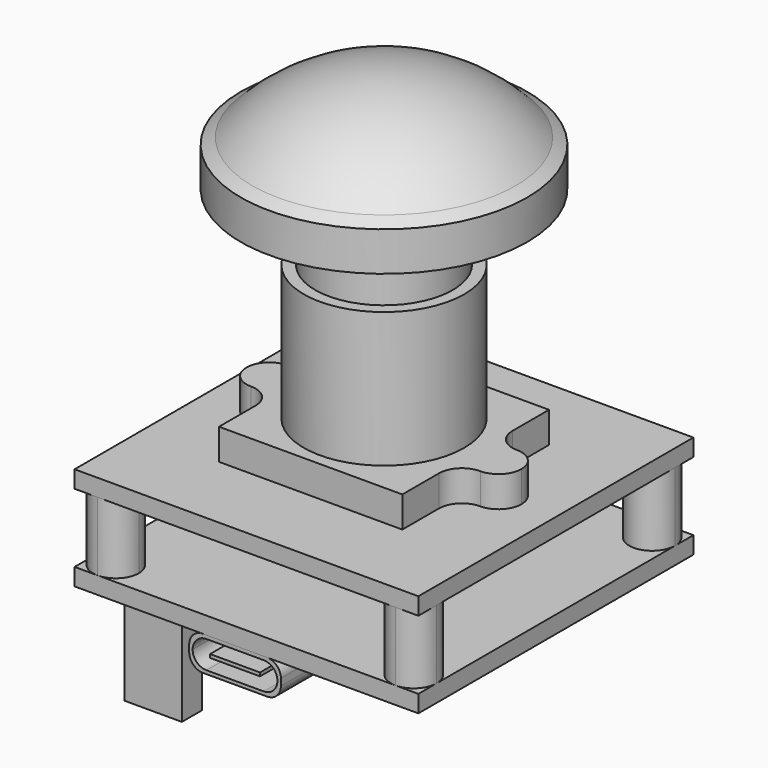
from build123d import *

# Parameters (mm, degrees)
F0_W      = 30
F0_H      = 30
F1_DEPTH  = 1.5
F2_START  = 6
F1_FACE_W = 30
F1_FACE_H = 30
F2_DEPTH  = 1.5
F3_R      = 1.25
F4_DEPTH  = 6
F5_W      = 4
F5_H      = 4
F5_R      = 7
F6_DEPTH  = 2.7
F7_R      = 1.99999
F8_DEPTH  = 14.5
F9_W      = 6
F9_H      = 1.5
F9_H_2    = 5
F12_W     = 8
F12_H     = 9
F13_DEPTH = 3
F14_W     = 7.4
F14_H     = 2.4
F14_W_2   = 4.36
F14_H_2   = 0.3
F15_DEPTH = 8
F16_R     = 1.19999
F17_W     = 5
F17_H     = 2.2
F18_DEPTH = 7.5


# Not quite as in the source:
# - a fillet or chamfer is up to 0.001 mm smaller than in the source, because OpenCascade refuses the exact size


with BuildPart() as f1:
    # F0 (on Top) → F1 (new body)
    with BuildSketch(Plane.XY):
        Rectangle(F0_W, F0_H)
    extrude(amount=F1_DEPTH)


with BuildPart() as f2:
    # F1_face (on face) → F2 (new body)
    with BuildSketch(Plane.XY.offset(1.5).offset(F2_START)):
        Rectangle(F1_FACE_W, F1_FACE_H)
    extrude(amount=F2_DEPTH)


with BuildPart() as f4:
    # F3 (on face) → F4 (new body)
    with BuildSketch(Plane.XY.offset(1.5)):
        with BuildLine():
            ThreePointArc((-11, 13), (-11.5857864376, 14.4142135624), (-13, 15))
            ThreePointArc((-13, 15), (-14.4142135624, 14.4142135624), (-15, 13))
            ThreePointArc((-15, 13), (-13, 11), (-11, 13))
        make_face()
        with Locations((-13, 13)):
            Circle(F3_R, mode=Mode.SUBTRACT)
    extrude(amount=F4_DEPTH)


with BuildPart() as f4b:
    # F3 (on face) → F4, piece 2 (new body)
    with BuildSketch(Plane.XY.offset(1.5)):
        with BuildLine():
            ThreePointArc((-15, -13), (-14.4142135624, -14.4142135624), (-13, -15))
            ThreePointArc((-13, -15), (-11.5857864376, -14.4142135624), (-11, -13))
            ThreePointArc((-11, -13), (-13, -11), (-15, -13))
        make_face()
        with Locations((-13, -13)):
            Circle(F3_R, mode=Mode.SUBTRACT)
    extrude(amount=F4_DEPTH)


with BuildPart() as f4c:
    # F3 (on face) → F4, piece 3 (new body)
    with BuildSketch(Plane.XY.offset(1.5)):
        with BuildLine():
            ThreePointArc((13, -15), (14.4142135624, -14.4142135624), (15, -13))
            ThreePointArc((15, -13), (11.5857864376, -11.5857864376), (13, -15))
        make_face()
        with Locations((13, -13)):
            Circle(F3_R, mode=Mode.SUBTRACT)
    extrude(amount=F4_DEPTH)


with BuildPart() as f4d:
    # F3 (on face) → F4, piece 4 (new body)
    with BuildSketch(Plane.XY.offset(1.5)):
        with BuildLine():
            ThreePointArc((13, 15), (11.5857864376, 11.5857864376), (15, 13))
            ThreePointArc((15, 13), (14.4142135624, 14.4142135624), (13, 15))
        make_face()
        with Locations((13, 13)):
            Circle(F3_R, mode=Mode.SUBTRACT)
    extrude(amount=F4_DEPTH)


with BuildPart() as f6:
    # F5 (on face) → F6 (new body)
    with BuildSketch(Plane.XY.offset(9)):
        with Locations((-10, 0)):
            Rectangle(F5_W, F5_H)
        Polygon((-8, -8), (8, -8), (8, -2), (8, 2), (8, 8), (-8, 8), (-8, 2), (-8, -2), align=None)
        Circle(F5_R, mode=Mode.SUBTRACT)
        with Locations((10, 0)):
            Rectangle(F5_W, F5_H)
        Circle(F5_R)
    extrude(amount=F6_DEPTH)

    # F7 (radius 2 in the source; OpenCascade refuses exactly that, so slightly less here)
    f7_edges = [f6.edges().sort_by_distance(p)[0] for p in [
        (-12, 2, 10.35),
        (-12, -2, 10.35),
        (-8, 2, 10.35),
        (-8, -2, 10.35),
        (12, -2, 10.35),
        (8, -2, 10.35),
        (8, 2, 10.35),
        (12, 2, 10.35),
    ]]
    fillet(f7_edges, radius=F7_R)

    # F5 (on face) → F8 (join)
    with BuildSketch(Plane.XY.offset(9)):
        Circle(F5_R)
    extrude(amount=F8_DEPTH)


with BuildPart() as f10:
    # F9 (on Front) → F10 (revolve)
    with BuildSketch(Plane.XZ):
        with BuildLine():
            Line((-11.5, 33.3), (0, 33.3))
            Line((0, 33.3), (0, 38.3))
            ThreePointArc((0, 38.3), (-6.269968102, 36.9959266346), (-11.5, 33.3))
        make_face()
    revolve(axis=Axis((0, 0, 25.3), (0, 0, -1)))


with BuildPart() as f11:
    # F9 (on Front) → F11 (revolve)
    with BuildSketch(Plane.XZ):
        Polygon((-6, 29.3), (0, 29.3), (0, 33.3), (-11.5, 33.3), (-12.5, 32.7226497308), (-12.5, 29.3), align=None)
        with Locations((-3, 28.55)):
            Rectangle(F9_W, F9_H)
        with Locations((-3, 25.3)):
            Rectangle(F9_W, F9_H_2)
    revolve(axis=Axis((0, 0, 25.3), (0, 0, -1)))


with BuildPart() as f13:
    # F12 (on face) → F13 (new body)
    with BuildSketch(Plane(origin=(0, 0, 0), x_dir=(1, 0, 0), z_dir=(0, 0, -1))):
        with Locations((-1, 10.5)):
            Rectangle(F12_W, F12_H)
    extrude(amount=F13_DEPTH)

    # F14 (on face) → F15 (cut)
    with BuildSketch(Plane.XZ.offset(15)):
        with Locations((-1, -1.5)):
            Rectangle(F14_W, F14_H)
        with Locations((-1, -1.5)):
            Rectangle(F14_W_2, F14_H_2, mode=Mode.SUBTRACT)
    extrude(amount=-F15_DEPTH, mode=Mode.SUBTRACT)

    # F16 (radius 1.2 in the source; OpenCascade refuses exactly that, so slightly less here)
    f16_edges = [f13.edges().sort_by_distance(p)[0] for p in [
        (-5, -10.5, -3),
        (-5, -10.5, 0),
        (3, -10.5, 0),
        (3, -10.5, -3),
        (-4.7, -11, -0.3),
        (2.7, -11, -0.3),
        (2.7, -11, -2.7),
        (-4.7, -11, -2.7),
    ]]
    fillet(f16_edges, radius=F16_R)


with BuildPart() as f18:
    # F17 (on face) → F18 (new body)
    with BuildSketch(Plane(origin=(0, 0, 0), x_dir=(1, 0, 0), z_dir=(0, 0, -1))):
        with Locations((-8.3, 13.7)):
            Rectangle(F17_W, F17_H)
    extrude(amount=F18_DEPTH)


solid = Compound([f1.part, f2.part, f4.part, f4b.part, f4c.part, f4d.part, f6.part, f10.part, f11.part, f13.part, f18.part])
